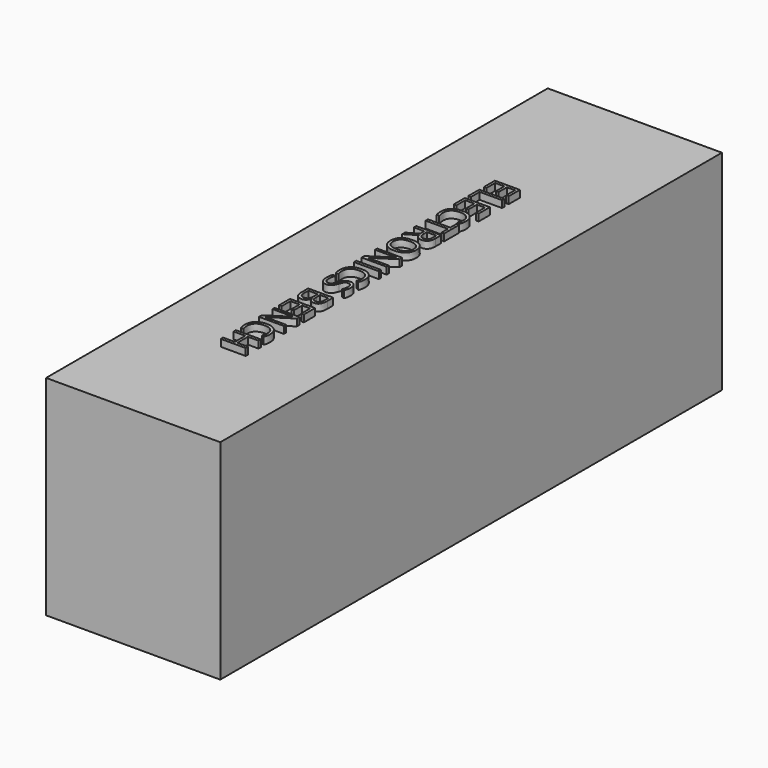
from build123d import *

# Parameters (mm, degrees)
F0_W         = 762
F0_H         = 2743.2
F1_DEPTH     = 914.4
F2_TEXT_SIZE = 152.7269310869
F3_DEPTH     = 30.48


# Not quite as in the source:
# - Text() gives the source's letters only with a copy of the font that has no kerning and outlines rounded to 1/6400 em; it was checked with that copy


with BuildPart() as f1:
    # F0 (on Top) → F1 (new body)
    with BuildSketch(Plane.XY):
        Rectangle(F0_W, F0_H)
    extrude(amount=F1_DEPTH)

    # F2 (on face) → F3 (join)
    with BuildSketch(Plane.XY.offset(914.4)):
        with Locations(Location((-58.7419331055, 694.849509324), (0, 0, -90))):
            Text('ELECTRONICS BENCH', F2_TEXT_SIZE, font='Open Sans', text_align=(TextAlign.LEFT, TextAlign.BOTTOM))
    extrude(amount=F3_DEPTH)


solid = f1.part
